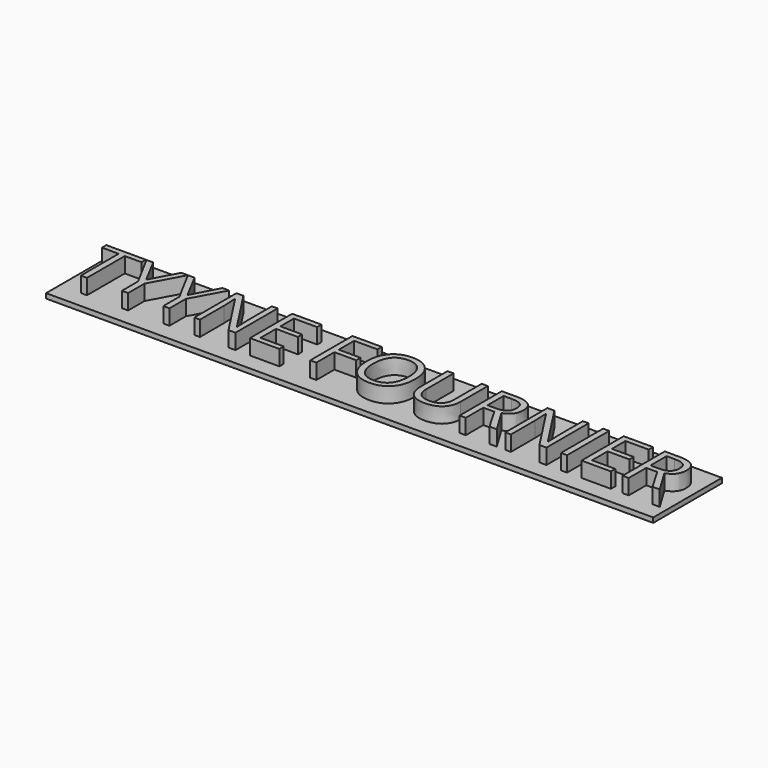
from build123d import *

# Parameters (mm, degrees)
F0_W         = 251.46
F0_H         = 35.5501176417
F1_DEPTH     = 2.00000108
F3_TEXT_SIZE = 30.5845492244
F4_DEPTH     = 6.35


# Not quite as in the source:
# - Text() gives the source's letters only with a copy of the font that has no kerning and outlines rounded to 1/6400 em; it was checked with that copy


with BuildPart() as f1:
    # F0 (on Top) → F1 (new body)
    with BuildSketch(Plane.XY):
        with Locations((-1.3476610184, 1.2259781361)):
            Rectangle(F0_W, F0_H)
    extrude(amount=F1_DEPTH)


with BuildPart() as f4:
    # F3 (on face) → F4 (new body)
    with BuildSketch(Plane.XY.offset(2.00000108)):
        with Locations((-125.5388169827, -9.4627952269)):
            Text('TYYNE FOURNIER', F3_TEXT_SIZE, font='Open Sans', text_align=(TextAlign.LEFT, TextAlign.BOTTOM))
    extrude(amount=F4_DEPTH)


solid = Compound([f1.part, f4.part])
